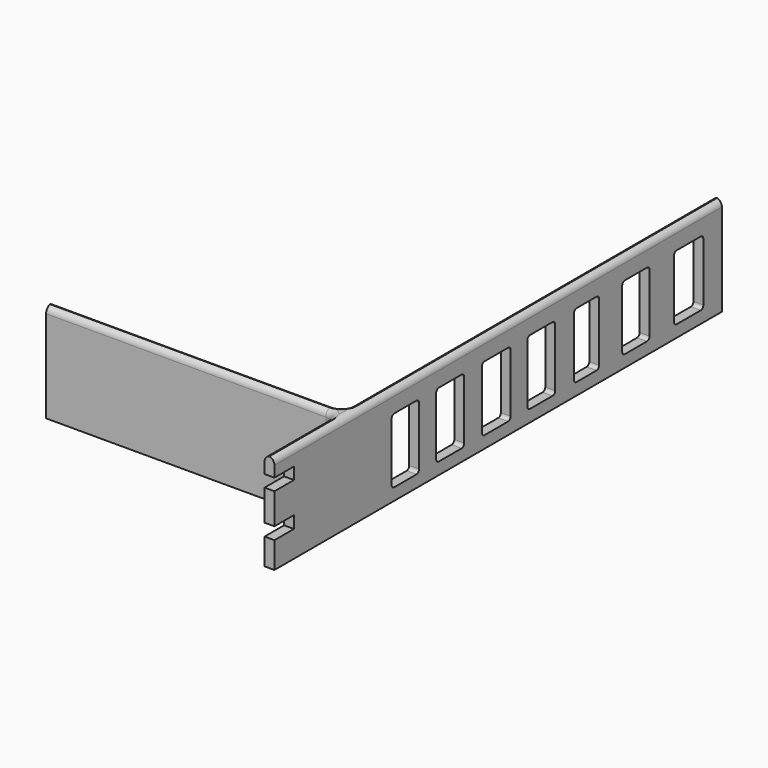
from build123d import *

# Parameters (mm, degrees)
F0_W         = 88
F0_H         = 3
F1_DEPTH     = 30
F2_R         = 3
F3_T1_DEPTH  = 142
F3_T3_DEPTH  = 90
F3_T5_DEPTH  = 180
F3_T7_DEPTH  = 29
F3_T10_ANGLE = 90
F3_T12_ANGLE = 90
F4_W         = 7.4076932669
F4_H         = 3.6282110959
F4_H_2       = 3.7070848048
F5_DEPTH     = 3
F6_W         = 11.1425933428
F6_H         = 19.764843164
F6_W_2       = 10.4046501219
F6_H_2       = 19.7511005681
F6_W_3       = 9.5925889909
F6_W_4       = 10.5412900448
F6_W_5       = 10.9199807048
F6_W_6       = 10.6662213802
F6_W_7       = 10.4241892695
F7_DEPTH     = 3
F8_R         = 1


# Not quite as in the source:
# - a fillet or chamfer that OpenCascade refuses, or shapes differently, is made with other operations: its cross-section is extruded or revolved along the edge and cut away or added


with BuildPart() as f1:
    # F0 (on Top) → F1 (new body)
    with BuildSketch(Plane.XY):
        Polygon((3, 0), (0, 0), (0, -140), (0, -143), (0, -170), (3, -170), (3, -140), align=None)
        with Locations((-44, -141.5)):
            Rectangle(F0_W, F0_H)
    extrude(amount=F1_DEPTH)

    # F2
    f2_edges = [f1.edges().sort_by_distance(p)[0] for p in [
        (0, -140, 15),
        (0, -143, 15),
    ]]
    fillet(f2_edges, radius=F2_R)

    # F3: fillet of radius 2 on 3 edges, made by hand

    # F3_s2 → F3_t1 (cut)
    with BuildSketch(Plane.XZ.offset(-5)):
        with BuildLine():
            ThreePointArc((0, 28), (0.5857864376, 29.4142135624), (2, 30))
            Line((2, 30), (0, 30))
            Line((0, 30), (0, 28))
        make_face()
    extrude(amount=F3_T1_DEPTH, mode=Mode.SUBTRACT)

    # F3_s4 → F3_t3 (cut)
    with BuildSketch(Plane.YZ.offset(-93)):
        with BuildLine():
            ThreePointArc((-141, 30), (-142.4142135624, 29.4142135624), (-143, 28))
            Line((-143, 28), (-143, 30))
            Line((-143, 30), (-141, 30))
        make_face()
        with BuildLine():
            ThreePointArc((-142, 30), (-140.5857864376, 29.4142135624), (-140, 28))
            Line((-140, 28), (-140, 30))
            Line((-140, 30), (-142, 30))
        make_face()
    extrude(amount=F3_T3_DEPTH, mode=Mode.SUBTRACT)

    # F3_s6 → F3_t5 (cut)
    with BuildSketch(Plane.XZ.offset(-5)):
        with BuildLine():
            ThreePointArc((1, 30), (2.4142135624, 29.4142135624), (3, 28))
            Line((3, 28), (3, 30))
            Line((3, 30), (1, 30))
        make_face()
    extrude(amount=F3_T5_DEPTH, mode=Mode.SUBTRACT)

    # F3_s8 → F3_t7 (cut)
    with BuildSketch(Plane.XZ.offset(146)):
        with BuildLine():
            ThreePointArc((2, 30), (0.5857864376, 29.4142135624), (0, 28))
            Line((0, 28), (0, 30))
            Line((0, 30), (2, 30))
        make_face()
    extrude(amount=F3_T7_DEPTH, mode=Mode.SUBTRACT)

    # F3_s9 → F3_t10 (revolve, cut)
    with BuildSketch(Plane.YZ.offset(-3)):
        with BuildLine():
            ThreePointArc((-141, 30), (-142.4142135624, 29.4142135624), (-143, 28))
            Line((-143, 28), (-143, 30))
            Line((-143, 30), (-141, 30))
        make_face()
    revolve(axis=Axis((-3, -146, 30), (0, 0, -1)), revolution_arc=F3_T10_ANGLE, mode=Mode.SUBTRACT)

    # F3_s11 → F3_t12 (revolve, cut)
    with BuildSketch(Plane.XZ.offset(137)):
        with BuildLine():
            ThreePointArc((0, 28), (0.5857864376, 29.4142135624), (2, 30))
            Line((2, 30), (0, 30))
            Line((0, 30), (0, 28))
        make_face()
    revolve(axis=Axis((-3, -137, 30), (0, 0, -1)), revolution_arc=F3_T12_ANGLE, mode=Mode.SUBTRACT)

    # F4 (on face) → F5 (cut)
    with BuildSketch(Plane(origin=(0, 0, 0), x_dir=(0, -1, 0), z_dir=(-1, 0, 0))):
        with Locations((166.2961533666, 22.8808587417)):
            Rectangle(F4_W, F4_H)
        with Locations((166.2961533666, 9.8271891475)):
            Rectangle(F4_W, F4_H_2)
    extrude(amount=-F5_DEPTH, mode=Mode.SUBTRACT)

    # F6 (on face) → F7 (cut)
    with BuildSketch(Plane(origin=(0, 0, 0), x_dir=(0, -1, 0), z_dir=(-1, 0, 0))):
        with Locations((12.6331185456, 13.5222995887)):
            Rectangle(F6_W, F6_H)
        with Locations((32.683422789, 13.5154282907)):
            Rectangle(F6_W_2, F6_H_2)
        with Locations((51.4230821282, 13.5154282907)):
            Rectangle(F6_W_3, F6_H_2)
        with Locations((68.6303824186, 13.5154282907)):
            Rectangle(F6_W_4, F6_H_2)
        with Locations((85.6932289898, 13.5154282907)):
            Rectangle(F6_W_5, F6_H_2)
        with Locations((103.2284647226, 13.5154282907)):
            Rectangle(F6_W_6, F6_H_2)
        with Locations((120.2503331006, 13.5154282907)):
            Rectangle(F6_W_7, F6_H_2)
    extrude(amount=-F7_DEPTH, mode=Mode.SUBTRACT)

    # F8
    f8_edges = [f1.edges().sort_by_distance(p)[0] for p in [
        (1.5, -7.061822, 23.404721),
        (1.5, -27.481098, 23.390979),
        (1.5, -46.626788, 23.390979),
        (1.5, -63.359737, 23.390979),
        (1.5, -80.233239, 23.390979),
        (1.5, -97.895354, 23.390979),
        (1.5, -115.038238, 23.390979),
        (1.5, -7.061822, 3.639878),
        (1.5, -27.481098, 3.639878),
        (1.5, -46.626788, 3.639878),
        (1.5, -63.359737, 3.639878),
        (1.5, -80.233239, 3.639878),
        (1.5, -97.895354, 3.639878),
        (1.5, -115.038238, 3.639878),
        (1.5, -125.462428, 23.390979),
        (1.5, -108.561575, 23.390979),
        (1.5, -91.153219, 23.390979),
        (1.5, -73.901027, 23.390979),
        (1.5, -56.219377, 23.390979),
        (1.5, -37.885748, 23.390979),
        (1.5, -18.204415, 23.404721),
        (1.5, -18.204415, 3.639878),
        (1.5, -37.885748, 3.639878),
        (1.5, -56.219377, 3.639878),
        (1.5, -73.901027, 3.639878),
        (1.5, -91.153219, 3.639878),
        (1.5, -108.561575, 3.639878),
        (1.5, -125.462428, 3.639878),
    ]]
    fillet(f8_edges, radius=F8_R)


solid = f1.part
